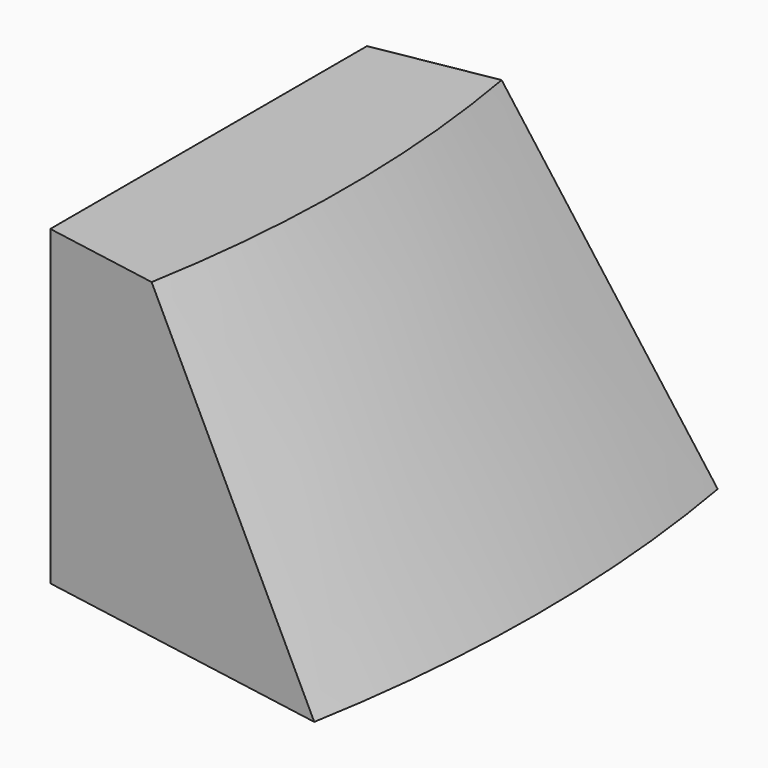
from build123d import *

# Parameters (mm, degrees)
F5_ANGLE_BACK = 10
F5_ANGLE      = 20
F3_DEPTH      = 15
F1_R          = 5
F4_DEPTH      = 61.9


with BuildPart() as f5:
    # F0 (on Front) → F5 (revolve)
    with BuildSketch(Plane.XZ, mode=Mode.PRIVATE) as f5_sk:
        Polygon((69.7967915205, 0), (60.5548890955, 15), (54.7967915205, 15), (54.7967915205, 0), align=None)
    revolve(f5_sk.sketch.rotate(Axis((0, 0, 12.625), (0, 0, 1)), -F5_ANGLE_BACK), axis=Axis((0, 0, 12.625), (0, 0, 1)), revolution_arc=F5_ANGLE)

    # F2 (on face) → F3 (join)
    with BuildSketch(Plane.XY.offset(15)):
        Polygon((54.7967915205, 9.6621528013), (53.9643051295, 9.5153629895), (53.9643051295, -9.5153629895), (54.7967915205, -9.6621528013), (56.5004897511, 0), align=None)
    extrude(amount=-F3_DEPTH)

    # F1 (on Right) → F4 (cut)
    with BuildSketch(Plane.YZ):
        with Locations((0, 7.5)):
            Circle(F1_R)
    extrude(amount=F4_DEPTH, mode=Mode.SUBTRACT)


solid = f5.part
